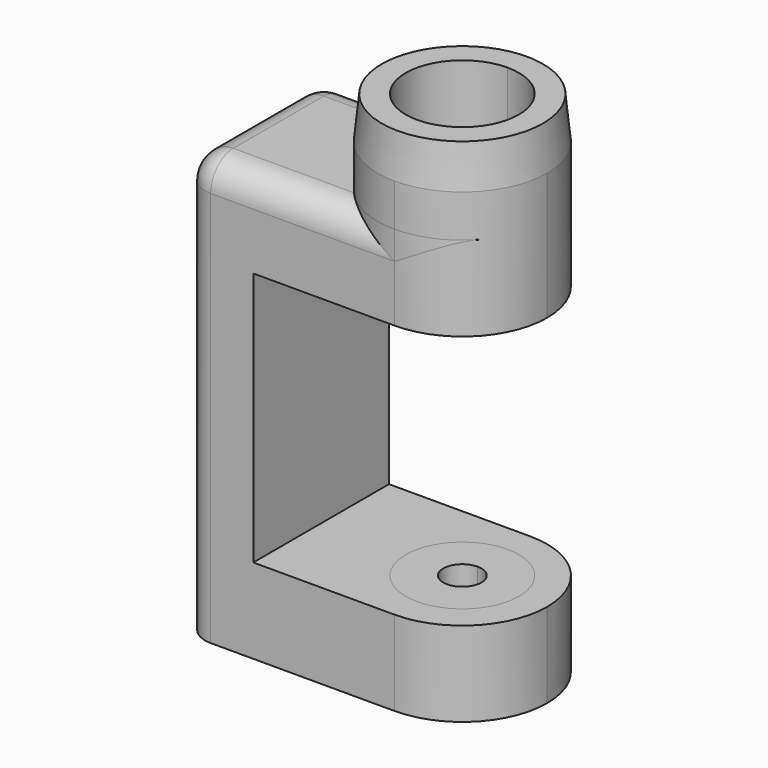
from build123d import *

# Parameters (mm, degrees)
F4_DEPTH     = 30
F5_DEPTH     = 36
F6_W         = 9.9882828072
F6_H         = 18
F6_W_2       = 6
F7_DEPTH     = 25
F1_DEPTH     = 25
F2_T1_DEPTH  = 8
F2_T6_DEPTH  = 18
F2_S7_R      = 6
F2_T8_DEPTH  = 11
F2_T12_DEPTH = 18
F2_S13_R     = 6
F2_T14_DEPTH = 11
F2_T16_ANGLE = 90
F2_T18_ANGLE = 90


# Not quite as in the source:
# - a fillet or chamfer that OpenCascade refuses, or shapes differently, is made with other operations: its cross-section is extruded or revolved along the edge and cut away or added


with BuildPart() as f4:
    # F3 (on Top) → F4 (new body)
    with BuildSketch(Plane.XY):
        with BuildLine():
            Line((0, 1.35), (0, 4))
            ThreePointArc((0, 4), (-4, 0), (0, -4))
            Line((0, -4), (0, -1.35))
            ThreePointArc((0, -1.35), (-1.35, 0), (0, 1.35))
        make_face()
        with BuildLine():
            ThreePointArc((4, 0), (2.8284271247, 2.8284271247), (0, 4))
            Line((0, 4), (0, 1.35))
            ThreePointArc((0, 1.35), (0.9545941546, 0.9545941546), (1.35, 0))
            ThreePointArc((1.35, 0), (0.9545941546, -0.9545941546), (0, -1.35))
            Line((0, -1.35), (0, -4))
            ThreePointArc((0, -4), (2.8284271247, -2.8284271247), (4, 0))
        make_face()
    extrude(amount=F4_DEPTH)


with BuildPart() as f4b:
    # F3 (on Top) → F4, piece 2 (new body)
    with BuildSketch(Plane.XY):
        with BuildLine():
            ThreePointArc((0, -6), (-6, 0), (0, 6))
            Line((0, 6), (-13, 6))
            ThreePointArc((-13, 6), (-14.4142135624, 5.4142135624), (-15, 4))
            Line((-15, 4), (-15, -4))
            ThreePointArc((-15, -4), (-14.4142135624, -5.4142135624), (-13, -6))
            Line((-13, -6), (0, -6))
        make_face()
    extrude(amount=F4_DEPTH)

    # F3 (on Top) → F5 (join)
    with BuildSketch(Plane.XY):
        with BuildLine():
            Line((0, 4), (0, 6))
            ThreePointArc((0, 6), (-6, 0), (0, -6))
            Line((0, -6), (0, -4))
            ThreePointArc((0, -4), (-4, 0), (0, 4))
        make_face()
        with BuildLine():
            ThreePointArc((0, -6), (4.2426406871, -4.2426406871), (6, 0))
            ThreePointArc((6, 0), (4.2426406871, 4.2426406871), (0, 6))
            Line((0, 6), (0, 4))
            ThreePointArc((0, 4), (2.8284271247, 2.8284271247), (4, 0))
            ThreePointArc((4, 0), (2.8284271247, -2.8284271247), (0, -4))
            Line((0, -4), (0, -6))
        make_face()
    extrude(amount=F5_DEPTH)

    # F0: chamfer of 3 x 0.3 on 1 edges, made by hand

    # F0_s1 → F0_t2 (revolve, cut)
    with BuildSketch(Plane.YZ):
        Polygon((-6, 33), (-5.7, 36), (-6, 36), align=None)
    revolve(axis=Axis((0, 0, 36), (0, 0, 1)), mode=Mode.SUBTRACT)


with BuildPart() as f7_tool:
    # F6 (on face) → F7 (new body)
    with BuildSketch(Plane.XZ.offset(6)):
        with Locations((-4.9941414036, 15)):
            Rectangle(F6_W, F6_H)
        with Locations((3, 15)):
            Rectangle(F6_W_2, F6_H)
    extrude(amount=-F7_DEPTH)


with BuildPart() as f4_1:
    add(f4.part)

    # F7: cut by f7_tool
    add(f7_tool.part, mode=Mode.SUBTRACT)

    # F6 (on face) → F1 (cut)
    with BuildSketch(Plane.XZ.offset(6)):
        with Locations((-4.9941414036, 15)):
            Rectangle(F6_W, F6_H)
        with Locations((3, 15)):
            Rectangle(F6_W_2, F6_H)
    extrude(amount=F1_DEPTH, mode=Mode.SUBTRACT)


with BuildPart() as f4b_1:
    add(f4b.part)

    # F7: cut by f7_tool
    add(f7_tool.part, mode=Mode.SUBTRACT)

    # F2: fillet of radius 2 on 5 edges, made by hand

    # F2_s2 → F2_t1 (cut)
    with BuildSketch(Plane.XZ.offset(-4)):
        with BuildLine():
            ThreePointArc((-15, 28), (-14.4142135624, 29.4142135624), (-13, 30))
            Line((-13, 30), (-15, 30))
            Line((-15, 30), (-15, 28))
        make_face()
    extrude(amount=F2_T1_DEPTH, mode=Mode.SUBTRACT)


with BuildPart() as f2_tool4:
    # F2_s5 → F2_t6 (new body)
    with BuildSketch(Plane.YZ.offset(5)):
        with BuildLine():
            ThreePointArc((6, 28), (5.4142135624, 29.4142135624), (4, 30))
            Line((4, 30), (6, 30))
            Line((6, 30), (6, 28))
        make_face()
    extrude(amount=-F2_T6_DEPTH)

    # F2_s7 → F2_t8 (cut, symmetric)
    with BuildSketch(Plane.XY.offset(29)):
        Circle(F2_S7_R)
    extrude(amount=F2_T8_DEPTH, both=True, mode=Mode.SUBTRACT)


with BuildPart() as f4b_2:
    add(f4b_1.part)

    # F2_t3: cut F2_tool4
    add(f2_tool4.part, mode=Mode.SUBTRACT)


with BuildPart() as f2_tool10:
    # F2_s11 → F2_t12 (new body)
    with BuildSketch(Plane.YZ.offset(-13)):
        with BuildLine():
            ThreePointArc((-6, 28), (-5.4142135624, 29.4142135624), (-4, 30))
            Line((-4, 30), (-6, 30))
            Line((-6, 30), (-6, 28))
        make_face()
    extrude(amount=F2_T12_DEPTH)

    # F2_s13 → F2_t14 (cut, symmetric)
    with BuildSketch(Plane.XY.offset(29)):
        Circle(F2_S13_R)
    extrude(amount=F2_T14_DEPTH, both=True, mode=Mode.SUBTRACT)


with BuildPart() as f4b_3:
    add(f4b_2.part)

    # F2_t9: cut F2_tool10
    add(f2_tool10.part, mode=Mode.SUBTRACT)

    # F2_s15 → F2_t16 (revolve, cut)
    with BuildSketch(Plane.XZ.offset(4)):
        with BuildLine():
            ThreePointArc((-15, 28), (-14.4142135624, 29.4142135624), (-13, 30))
            Line((-13, 30), (-15, 30))
            Line((-15, 30), (-15, 28))
        make_face()
    revolve(axis=Axis((-13, -4, 30), (0, 0, 1)), revolution_arc=F2_T16_ANGLE, mode=Mode.SUBTRACT)

    # F2_s17 → F2_t18 (revolve, cut)
    with BuildSketch(Plane.YZ.offset(-13)):
        with BuildLine():
            ThreePointArc((4, 30), (5.4142135624, 29.4142135624), (6, 28))
            Line((6, 28), (6, 30))
            Line((6, 30), (4, 30))
        make_face()
    revolve(axis=Axis((-13, 4, 30), (0, 0, 1)), revolution_arc=F2_T18_ANGLE, mode=Mode.SUBTRACT)


solid = Compound([f4_1.part, f4b_3.part])
